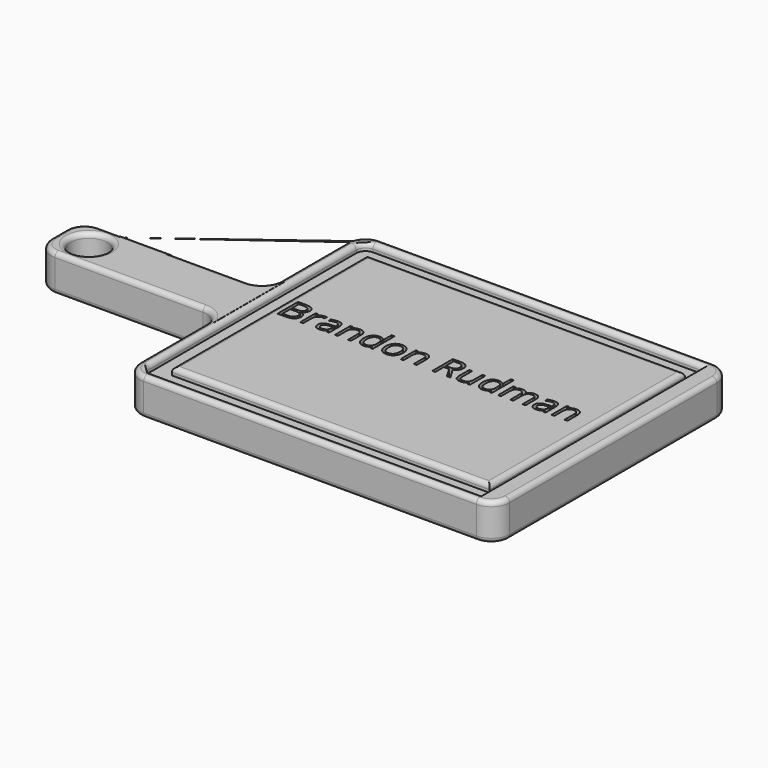
from build123d import *

# Parameters (mm, degrees)
F0_W         = 37.1430014968
F0_H         = 0.5493164063
F1_DEPTH     = 25.4
F2_R         = 12.7
F3_DEPTH     = 25.4
F5_DEPTH     = 5.08
F6_R         = 6.35
F7_R         = 12.7
F8_R         = 3.17499
F9_TEXT_SIZE = 24.6433714849
F10_DEPTH    = 5.08


# Not quite as in the source:
# - a fillet or chamfer is up to 0.001 mm smaller than in the source, because OpenCascade refuses the exact size
# - Text() gives the source's letters only with a copy of the font that has no kerning and outlines rounded to 1/6400 em; it was checked with that copy


with BuildPart() as f1:
    # F0 (on Top) → F1 (new body)
    with BuildSketch(Plane.XY):
        with Locations((-82.0715007484, 120.9246582031)):
            Rectangle(F0_W, F0_H)
        Polygon((-127, 82.55), (0, 82.55), (0, 120.65), (-63.5, 120.65), (-100.6430014968, 120.65), (-127, 120.65), align=None)
        Polygon((0, 82.55), (0, 0), (254, 0), (254, 203.2), (0, 203.2), (0, 120.65), align=None)
    extrude(amount=F1_DEPTH)

    # F2 (on face) → F3 (cut)
    with BuildSketch(Plane.XY.offset(25.4)):
        with Locations((-106.2270998955, 101.6)):
            Circle(F2_R)
    extrude(amount=-F3_DEPTH, mode=Mode.SUBTRACT)

    # F4 (on face) → F5 (cut)
    with BuildSketch(Plane.XY.offset(25.4)):
        Polygon((6.35, 82.55), (6.35, 6.35), (247.65, 6.35), (247.65, 196.85), (6.35, 196.85), (6.35, 120.65), align=None)
        Polygon((236.2200065136, 185.4200065136), (236.2200065136, 17.7799934864), (17.7799934864, 17.7799934864), (17.7799934864, 82.55), (17.7799934864, 120.65), (17.7799934864, 185.4200065136), align=None, mode=Mode.SUBTRACT)
    extrude(amount=-F5_DEPTH, mode=Mode.SUBTRACT)

    # F6
    f6_edges = [f1.edges().sort_by_distance(p)[0] for p in [
        (6.35, 196.85, 22.86),
        (247.65, 196.85, 22.86),
        (247.65, 6.35, 22.86),
        (6.35, 6.35, 22.86),
    ]]
    fillet(f6_edges, radius=F6_R)

    # F7
    f7_edges = [f1.edges().sort_by_distance(p)[0] for p in [
        (0, 0, 12.7),
        (-127, 82.55, 12.7),
        (-127, 120.65, 12.7),
        (0, 203.2, 12.7),
        (0, 120.65, 12.7),
        (0, 82.55, 12.7),
        (254, 203.2, 12.7),
        (254, 0, 12.7),
    ]]
    fillet(f7_edges, radius=F7_R)

    # F8 (radius 3.175 in the source; OpenCascade refuses exactly that, so slightly less here)
    f8_edges = [f1.edges().sort_by_distance(p)[0] for p in [
        (127, 185.420007, 25.4),
        (236.220007, 101.6, 25.4),
        (127, 17.779993, 25.4),
        (17.779993, 101.6, 25.4),
        (-38.1, 120.65, 25.4),
        (-3.719744, 124.369744, 25.4),
        (-63.5, 120.924658, 25.4),
        (0, 161.925, 25.4),
        (-82.071501, 121.199316, 25.4),
        (3.719744, 199.480256, 25.4),
        (-100.643001, 120.924658, 25.4),
        (127, 203.2, 25.4),
        (-107.471501, 120.65, 25.4),
        (250.280256, 199.480256, 25.4),
        (-123.280256, 116.930256, 25.4),
        (254, 101.6, 25.4),
        (-127, 101.6, 25.4),
        (250.280256, 3.719744, 25.4),
        (-123.280256, 86.269744, 25.4),
        (127, 0, 25.4),
        (-63.5, 82.55, 25.4),
        (3.719744, 3.719744, 25.4),
        (-3.719744, 78.830256, 25.4),
        (0, 41.275, 25.4),
        (127, 6.35, 25.4),
        (8.209872, 8.209872, 25.4),
        (245.790128, 8.209872, 25.4),
        (6.35, 101.6, 25.4),
        (247.65, 101.6, 25.4),
        (8.209872, 194.990128, 25.4),
        (245.790128, 194.990128, 25.4),
        (127, 196.85, 25.4),
        (-118.9271, 101.6, 25.4),
        (-38.1, 120.65, 0),
        (-3.719744, 124.369744, 0),
        (-63.5, 120.924658, 0),
        (0, 161.925, 0),
        (-82.071501, 121.199316, 0),
        (3.719744, 199.480256, 0),
        (-100.643001, 120.924658, 0),
        (127, 203.2, 0),
        (-107.471501, 120.65, 0),
        (250.280256, 199.480256, 0),
        (-123.280256, 116.930256, 0),
        (254, 101.6, 0),
        (-127, 101.6, 0),
        (250.280256, 3.719744, 0),
        (-123.280256, 86.269744, 0),
        (127, 0, 0),
        (-63.5, 82.55, 0),
        (3.719744, 3.719744, 0),
        (-3.719744, 78.830256, 0),
        (0, 41.275, 0),
        (-118.9271, 101.6, 0),
    ]]
    fillet(f8_edges, radius=F8_R)

    # F9 (on face) → F10 (cut)
    with BuildSketch(Plane.XY.offset(25.4)):
        with Locations((20.9549934864, 101.6)):
            Text('Brandon Rudman', F9_TEXT_SIZE, font='Open Sans', text_align=(TextAlign.LEFT, TextAlign.BOTTOM))
    extrude(amount=-F10_DEPTH, mode=Mode.SUBTRACT)


solid = f1.part
